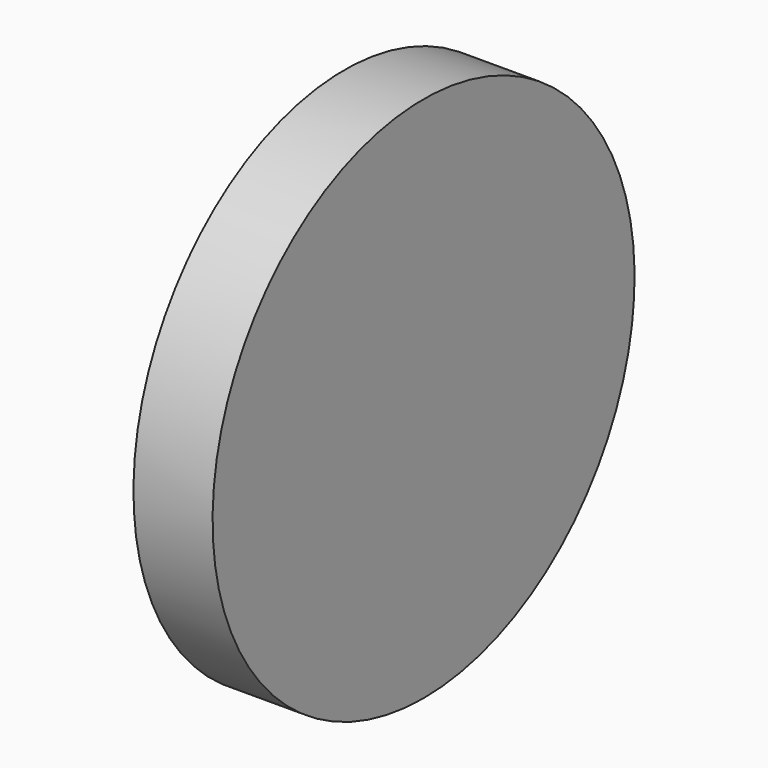
from build123d import *


# Not quite as in the source:
# - a feature of the source that left no trace in its solid (it failed there, or was rolled back) is left out


with BuildPart() as f1:
    # F0 (on Front) → F1 (revolve)
    with BuildSketch(Plane.XZ):
        with BuildLine():
            Line((-15.24, 0), (0, 0))
            Line((0, 0), (0, 50.8))
            Line((0, 50.8), (-6.35, 50.8))
            Line((-6.35, 50.8), (-4.7617064118, 41.792339449))
            ThreePointArc((-4.7617064118, 41.792339449), (-4.8311637627, 41.5331210865), (-5.0743828734, 41.4197061526))
            Line((-5.0743828734, 41.4197061526), (-6.2835011077, 41.4197061526))
            ThreePointArc((-6.2835011077, 41.4197061526), (-6.5080075107, 41.3267125556), (-6.6010011077, 41.1022061526))
            Line((-6.6010011077, 41.1022061526), (-6.6010011077, 40.4672061526))
            ThreePointArc((-6.6010011077, 40.4672061526), (-6.5080075107, 40.2426997495), (-6.2835011077, 40.1497061526))
            Line((-6.2835011077, 40.1497061526), (-5.0743828734, 40.1497061526))
            ThreePointArc((-5.0743828734, 40.1497061526), (-4.8311637627, 40.0362912186), (-4.7617064118, 39.7770728561))
            Line((-4.7617064118, 39.7770728561), (-5.2010717431, 37.2853082403))
            ThreePointArc((-5.2010717431, 37.2853082403), (-5.3096631386, 37.0972224261), (-5.5137482047, 37.0229415367))
            Line((-5.5137482047, 37.0229415367), (-6.8348340718, 37.0229415367))
            ThreePointArc((-6.8348340718, 37.0229415367), (-7.0593404748, 36.9299479398), (-7.1523340718, 36.7054415367))
            Line((-7.1523340718, 36.7054415367), (-7.1523340718, 36.0704415367))
            ThreePointArc((-7.1523340718, 36.0704415367), (-7.2453276688, 35.8459351337), (-7.4698340718, 35.7529415367))
            Line((-7.4698340718, 35.7529415367), (-8.7398340718, 35.7529415367))
            ThreePointArc((-8.7398340718, 35.7529415367), (-8.9643404748, 35.6599479398), (-9.0573340718, 35.4354415367))
            Line((-9.0573340718, 35.4354415367), (-9.0573340718, 34.8004415367))
            ThreePointArc((-9.0573340718, 34.8004415367), (-8.9643404748, 34.5759351337), (-8.7398340718, 34.4829415367))
            Line((-8.7398340718, 34.4829415367), (-3.5686493249, 34.4829415367))
            ThreePointArc((-3.5686493249, 34.4829415367), (-3.3254302142, 34.3695266028), (-3.2559728633, 34.1103082403))
            Line((-3.2559728633, 34.1103082403), (-7.113602572, 12.2326030065))
            ThreePointArc((-7.113602572, 12.2326030065), (-7.2221939675, 12.0445171922), (-7.4262790336, 11.9702363029))
            Line((-7.4262790336, 11.9702363029), (-8.1123649007, 11.9702363029))
            ThreePointArc((-8.1123649007, 11.9702363029), (-8.3368713037, 11.8772427059), (-8.4298649007, 11.6527363029))
            Line((-8.4298649007, 11.6527363029), (-8.4298649007, 8.9432889844))
            ThreePointArc((-8.4298649007, 8.9432889844), (-8.4596121783, 8.8091076862), (-8.5432798346, 8.7000698737))
            Line((-8.5432798346, 8.7000698737), (-15.1265850661, 3.176020882))
            ThreePointArc((-15.1265850661, 3.176020882), (-15.2102527224, 3.0669830694), (-15.24, 2.9328017713))
            Line((-15.24, 2.9328017713), (-15.24, 0))
        make_face()
    revolve(axis=Axis((-3.175, 0, 50.8), (-1, 0, 0)))


solid = f1.part
